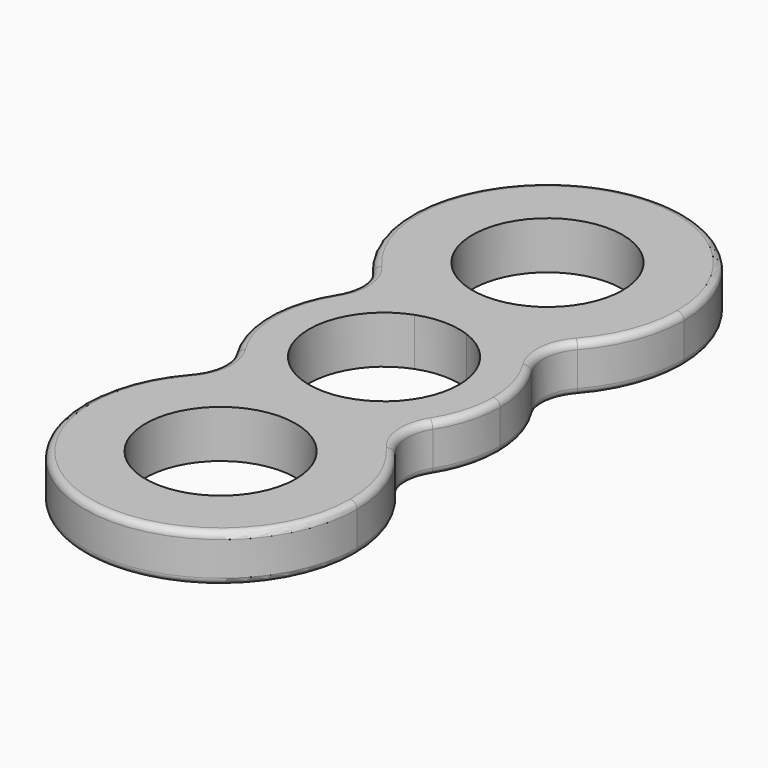
from build123d import *

# Parameters (mm, degrees)
F0_R     = 11.025
F1_DEPTH = 7
F2_R     = 1


# Not quite as in the source:
# - a feature names something its author has since deleted; it is built from what else it names


with BuildPart() as f1:
    # F0 (on Top) → F1 (new body)
    with BuildSketch(Plane.XY):
        with BuildLine():
            ThreePointArc((3.8188111697, 10.3425), (9.045800632, 6.3027070317), (11.025, 0))
            ThreePointArc((11.025, 0), (9.045800632, -6.3027070317), (3.8188111697, -10.3425))
            ThreePointArc((3.8188111697, -10.3425), (7.4507812466, -11.4127332882), (10.8163704055, -13.1475))
            ThreePointArc((10.8163704055, -13.1475), (12.7757955184, -11.2529851094), (14.4077918935, -9.0700693357))
            ThreePointArc((14.4077918935, -9.0700693357), (16.3576172162, -4.7200618647), (17.025, 0))
            ThreePointArc((17.025, 0), (16.3576172162, 4.7200618647), (14.4077918935, 9.0700693357))
            ThreePointArc((14.4077918935, 9.0700693357), (12.7757955184, 11.2529851094), (10.8163704055, 13.1475))
            ThreePointArc((10.8163704055, 13.1475), (7.4507812466, 11.4127332882), (3.8188111697, 10.3425))
        make_face()
        with BuildLine():
            ThreePointArc((-3.8188111697, -10.3425), (-11.025, 0), (-3.8188111697, 10.3425))
            ThreePointArc((-3.8188111697, 10.3425), (-7.4507812466, 11.4127332882), (-10.8163704055, 13.1475))
            ThreePointArc((-10.8163704055, 13.1475), (-12.7757955184, 11.2529851094), (-14.4077918935, 9.0700693357))
            ThreePointArc((-14.4077918935, 9.0700693357), (-17.025, 0), (-14.4077918935, -9.0700693357))
            ThreePointArc((-14.4077918935, -9.0700693357), (-12.7757955184, -11.2529851094), (-10.8163704055, -13.1475))
            ThreePointArc((-10.8163704055, -13.1475), (-7.4507812466, -11.4127332882), (-3.8188111697, -10.3425))
        make_face()
        with BuildLine():
            ThreePointArc((-10.8163704055, 13.1475), (0, 17.025), (10.8163704055, 13.1475))
            ThreePointArc((10.8163704055, 13.1475), (13.0469549327, 14.808634295), (15.0258776109, 16.7627938362))
            ThreePointArc((15.0258776109, 16.7627938362), (18.7335771298, 22.9251351305), (20.025, 30))
            ThreePointArc((20.025, 30), (-7.0748648695, 48.7335771298), (-15.0258776109, 16.7627938362))
            ThreePointArc((-15.0258776109, 16.7627938362), (-13.0469549327, 14.808634295), (-10.8163704055, 13.1475))
        make_face()
        with Locations((0, 30)):
            Circle(F0_R, mode=Mode.SUBTRACT)
        with BuildLine():
            ThreePointArc((15.0258776109, 16.7627938362), (13.0469549327, 14.808634295), (10.8163704055, 13.1475))
            ThreePointArc((10.8163704055, 13.1475), (12.7757955184, 11.2529851094), (14.4077918935, 9.0700693357))
            ThreePointArc((14.4077918935, 9.0700693357), (13.4378751676, 13.0191918827), (15.0258776109, 16.7627938362))
        make_face()
        with BuildLine():
            ThreePointArc((15.0258776109, -16.7627938362), (13.0469549327, -14.808634295), (10.8163704055, -13.1475))
            ThreePointArc((10.8163704055, -13.1475), (0, -17.025), (-10.8163704055, -13.1475))
            ThreePointArc((-10.8163704055, -13.1475), (-13.0469549327, -14.808634295), (-15.0258776109, -16.7627938362))
            ThreePointArc((-15.0258776109, -16.7627938362), (-7.0748648695, -48.7335771298), (20.025, -30))
            ThreePointArc((20.025, -30), (18.7335771298, -22.9251351305), (15.0258776109, -16.7627938362))
        make_face()
        with Locations((0, -30)):
            Circle(F0_R, mode=Mode.SUBTRACT)
        with BuildLine():
            ThreePointArc((14.4077918935, -9.0700693357), (12.7757955184, -11.2529851094), (10.8163704055, -13.1475))
            ThreePointArc((10.8163704055, -13.1475), (13.0469549327, -14.808634295), (15.0258776109, -16.7627938362))
            ThreePointArc((15.0258776109, -16.7627938362), (13.4378751676, -13.0191918827), (14.4077918935, -9.0700693357))
        make_face()
        with BuildLine():
            ThreePointArc((-14.4077918935, 9.0700693357), (-12.7757955184, 11.2529851094), (-10.8163704055, 13.1475))
            ThreePointArc((-10.8163704055, 13.1475), (-13.0469549327, 14.808634295), (-15.0258776109, 16.7627938362))
            ThreePointArc((-15.0258776109, 16.7627938362), (-13.4378751676, 13.0191918827), (-14.4077918935, 9.0700693357))
        make_face()
        with BuildLine():
            ThreePointArc((-15.0258776109, -16.7627938362), (-13.0469549327, -14.808634295), (-10.8163704055, -13.1475))
            ThreePointArc((-10.8163704055, -13.1475), (-12.7757955184, -11.2529851094), (-14.4077918935, -9.0700693357))
            ThreePointArc((-14.4077918935, -9.0700693357), (-13.4378751676, -13.0191918827), (-15.0258776109, -16.7627938362))
        make_face()
        with BuildLine():
            ThreePointArc((-3.8188111697, 10.3425), (0, 11.025), (3.8188111697, 10.3425))
            ThreePointArc((3.8188111697, 10.3425), (7.4507812466, 11.4127332882), (10.8163704055, 13.1475))
            ThreePointArc((10.8163704055, 13.1475), (0, 17.025), (-10.8163704055, 13.1475))
            ThreePointArc((-10.8163704055, 13.1475), (-7.4507812466, 11.4127332882), (-3.8188111697, 10.3425))
        make_face()
        with BuildLine():
            ThreePointArc((10.8163704055, -13.1475), (7.4507812466, -11.4127332882), (3.8188111697, -10.3425))
            ThreePointArc((3.8188111697, -10.3425), (0, -11.025), (-3.8188111697, -10.3425))
            ThreePointArc((-3.8188111697, -10.3425), (-7.4507812466, -11.4127332882), (-10.8163704055, -13.1475))
            ThreePointArc((-10.8163704055, -13.1475), (0, -17.025), (10.8163704055, -13.1475))
        make_face()
    extrude(amount=F1_DEPTH)

    # F2
    f2_edges = [f1.edges().sort_by_distance(p)[0] for p in [
        (15.025878, 16.762794, 3.5),
        (-15.025878, 16.762794, 3.5),
        (0, 50.025, 0),
        (0, 50.025, 7),
        (-14.407792, 9.070069, 3.5),
        (-13.437875, 13.019192, 0),
        (-13.437875, 13.019192, 7),
        (-14.407792, -9.070069, 3.5),
        (-15.025878, -16.762794, 3.5),
        (-13.437875, -13.019192, 0),
        (-13.437875, -13.019192, 7),
        (15.025878, -16.762794, 3.5),
        (0, -50.025, 0),
        (0, -50.025, 7),
    ]]
    fillet(f2_edges, radius=F2_R)


solid = f1.part
